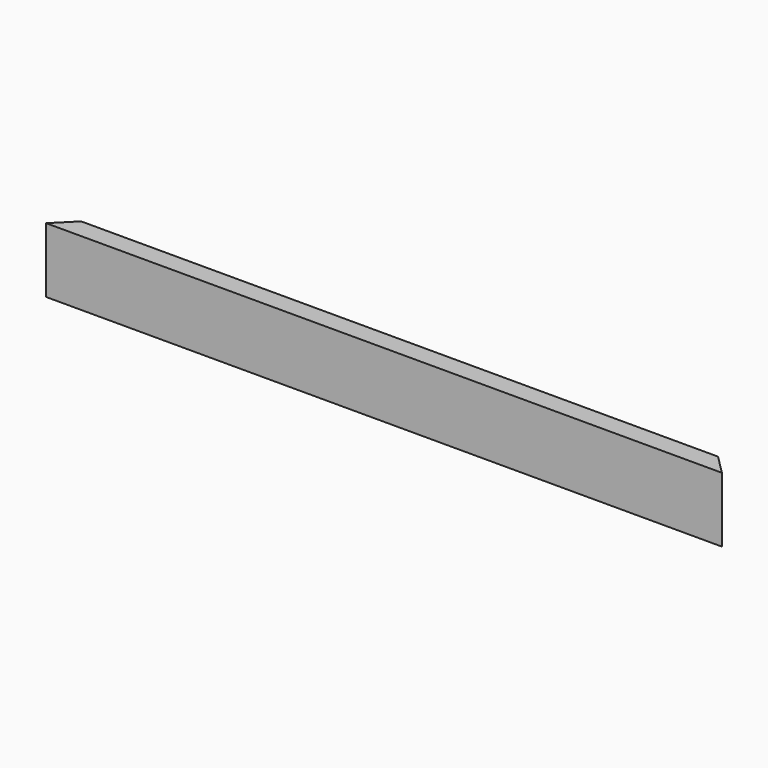
from build123d import *

# Parameters (mm, degrees)
F0_W     = 660.4
F0_H     = 63.5
F1_DEPTH = 19.05
F2_SIZE  = 19.04999


# Not quite as in the source:
# - a fillet or chamfer is up to 0.001 mm smaller than in the source, because OpenCascade refuses the exact size


with BuildPart() as f1:
    # F0 (on Front) → F1 (new body)
    with BuildSketch(Plane.XZ):
        with Locations((215.4097168565, -31.75)):
            Rectangle(F0_W, F0_H)
    extrude(amount=F1_DEPTH)

    # F2 (size 19.05 in the source; OpenCascade refuses exactly that, so slightly less here)
    f2_edges = [f1.edges().sort_by_distance(p)[0] for p in [
        (-114.790283, 0, -31.75),
        (545.609717, 0, -31.75),
    ]]
    chamfer(f2_edges, length=F2_SIZE)


solid = f1.part
